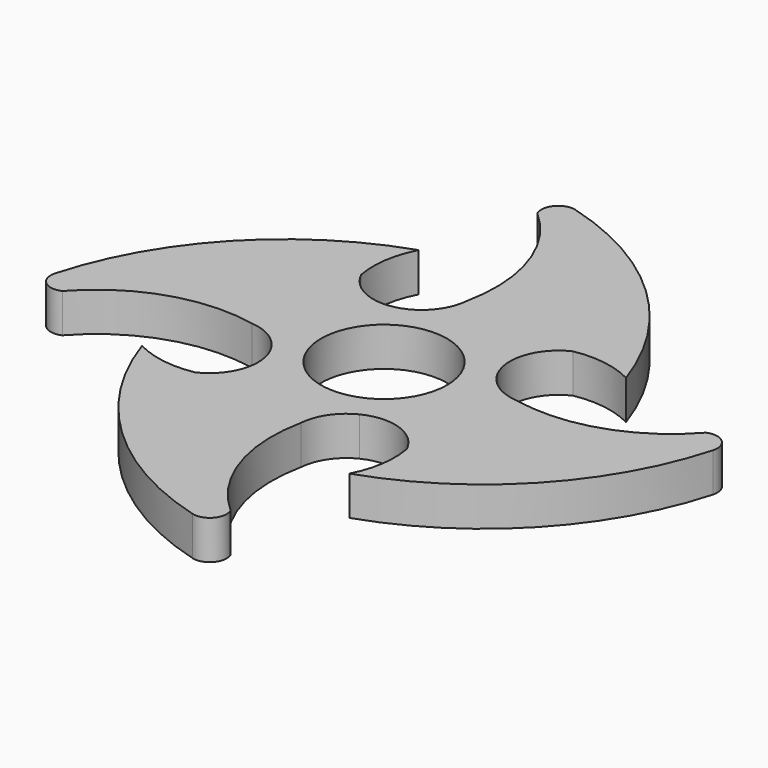
from build123d import *

# Parameters (mm, degrees)
F0_R        = 11.3
F1_DEPTH    = 7
F2_T1_DEPTH = 55.4992808982


# Not quite as in the source:
# - a fillet or chamfer that OpenCascade refuses, or shapes differently, is made with other operations: its cross-section is extruded or revolved along the edge and cut away or added
# - a feature names something its author has since deleted; it is built from what else it names


with BuildPart() as f1:
    # F0 (on Top) → F1 (new body)
    with BuildSketch(Plane.XY):
        with BuildLine():
            ThreePointArc((-19.0188516855, 18.6660698042), (-19.106601179, 24.2218879742), (-17.3798078978, 29.5032704141))
            ThreePointArc((-17.3798078978, 29.5032704141), (-42.8794362662, 11.5553714496), (-54.5032704141, -17.3798078978))
            ThreePointArc((-54.5032704141, -17.3798078978), (-51.6509498036, -14.2819027835), (-48.6055213036, -11.3736190606))
            ThreePointArc((-48.6055213036, -11.3736190606), (-36.3546417903, -3.2999675651), (-21.7060170396, -2.4719034169))
            ThreePointArc((-21.7060170396, -2.4719034169), (-17.5157178103, -3.9318400494), (-14.5899419176, -7.2679842351))
            ThreePointArc((-14.5899419176, -7.2679842351), (-15.4558877949, 5.1774059597), (-7.2679841768, 14.5899419466))
            ThreePointArc((-7.2679841768, 14.5899419466), (-14.000366861, 14.1575501664), (-19.0188516855, 18.6660698042))
        make_face()
        with BuildLine():
            ThreePointArc((-2.4719034169, 21.7060170396), (-3.9318400312, 17.5157178373), (-7.2679841768, 14.5899419466))
            ThreePointArc((-7.2679841768, 14.5899419466), (5.177405829, 15.4558878387), (14.5899417947, 7.2679844819))
            ThreePointArc((14.5899417947, 7.2679844819), (14.1575502222, 14.000367022), (18.6660698042, 19.0188516855))
            ThreePointArc((18.6660698042, 19.0188516855), (24.2218879742, 19.106601179), (29.5032704141, 17.3798078978))
            ThreePointArc((29.5032704141, 17.3798078978), (11.5553714496, 42.8794362662), (-17.3798078978, 54.5032704141))
            ThreePointArc((-17.3798078978, 54.5032704141), (-14.2819027835, 51.6509498036), (-11.3736190606, 48.6055213036))
            ThreePointArc((-11.3736190606, 48.6055213036), (-3.2999675651, 36.3546417903), (-2.4719034169, 21.7060170396))
        make_face()
        with BuildLine():
            ThreePointArc((14.5899417947, 7.2679844819), (5.177405829, 15.4558878387), (-7.2679841768, 14.5899419466))
            ThreePointArc((-7.2679841768, 14.5899419466), (-15.4558877949, 5.1774059597), (-14.5899419176, -7.2679842351))
            ThreePointArc((-14.5899419176, -7.2679842351), (-5.1774060707, -15.4558877577), (7.2679839673, -14.589942051))
            ThreePointArc((7.2679839673, -14.589942051), (13.8592593357, -8.5796812684), (16.3, 0))
            ThreePointArc((16.3, 0), (15.8667269979, 3.733225733), (14.5899417947, 7.2679844819))
        make_face()
        Circle(F0_R, mode=Mode.SUBTRACT)
        with BuildLine():
            ThreePointArc((7.2679839673, -14.589942051), (-5.1774060707, -15.4558877577), (-14.5899419176, -7.2679842351))
            ThreePointArc((-14.5899419176, -7.2679842351), (-14.157550177, -14.0003668918), (-18.6660698042, -19.0188516855))
            ThreePointArc((-18.6660698042, -19.0188516855), (-24.2218879742, -19.106601179), (-29.5032704141, -17.3798078978))
            ThreePointArc((-29.5032704141, -17.3798078978), (-11.5553714496, -42.8794362662), (17.3798078978, -54.5032704141))
            ThreePointArc((17.3798078978, -54.5032704141), (14.2819027835, -51.6509498036), (11.3736190606, -48.6055213036))
            ThreePointArc((11.3736190606, -48.6055213036), (3.2999675651, -36.3546417903), (2.4719034169, -21.7060170396))
            ThreePointArc((2.4719034169, -21.7060170396), (3.9318399658, -17.5157179344), (7.2679839673, -14.589942051))
        make_face()
        with BuildLine():
            ThreePointArc((21.7060170396, 2.4719034169), (17.515717696, 3.9318401265), (14.5899417947, 7.2679844819))
            ThreePointArc((14.5899417947, 7.2679844819), (15.8667269979, 3.733225733), (16.3, 0))
            ThreePointArc((16.3, 0), (13.8592593357, -8.5796812684), (7.2679839673, -14.589942051))
            ThreePointArc((7.2679839673, -14.589942051), (14.0003667504, -14.157550128), (19.0188516855, -18.6660698042))
            ThreePointArc((19.0188516855, -18.6660698042), (19.106601179, -24.2218879742), (17.3798078978, -29.5032704141))
            ThreePointArc((17.3798078978, -29.5032704141), (42.8794362662, -11.5553714496), (54.5032704141, 17.3798078978))
            ThreePointArc((54.5032704141, 17.3798078978), (51.6509498036, 14.2819027835), (48.6055213036, 11.3736190606))
            ThreePointArc((48.6055213036, 11.3736190606), (36.3546417903, 3.2999675651), (21.7060170396, 2.4719034169))
        make_face()
    extrude(amount=F1_DEPTH)

    # F2: fillet of radius 3 on 4 edges, made by hand

    # F2_s2 → F2_t1 (cut)
    with BuildSketch(Plane.XY.offset(-24.2496404491)):
        with BuildLine():
            ThreePointArc((-52.7416075724, -7.8412674467), (-51.7993975119, -10.9256989731), (-48.6055213036, -11.3736190606))
            ThreePointArc((-48.6055213036, -11.3736190606), (-51.6509498036, -14.2819027835), (-54.5032704141, -17.3798078978))
            ThreePointArc((-54.5032704141, -17.3798078978), (-53.8333652751, -12.5715819227), (-52.7416075724, -7.8412674467))
        make_face()
        with BuildLine():
            ThreePointArc((7.8412674467, -52.7416075724), (10.9256989731, -51.7993975119), (11.3736190606, -48.6055213036))
            ThreePointArc((11.3736190606, -48.6055213036), (14.2819027835, -51.6509498036), (17.3798078978, -54.5032704141))
            ThreePointArc((17.3798078978, -54.5032704141), (12.5715819227, -53.8333652751), (7.8412674467, -52.7416075724))
        make_face()
        with BuildLine():
            ThreePointArc((52.7416075724, 7.8412674467), (51.7993975119, 10.9256989731), (48.6055213036, 11.3736190606))
            ThreePointArc((48.6055213036, 11.3736190606), (51.6509498036, 14.2819027835), (54.5032704141, 17.3798078978))
            ThreePointArc((54.5032704141, 17.3798078978), (53.8333652751, 12.5715819227), (52.7416075724, 7.8412674467))
        make_face()
        with BuildLine():
            ThreePointArc((-7.8412674467, 52.7416075724), (-10.9256989731, 51.7993975119), (-11.3736190606, 48.6055213036))
            ThreePointArc((-11.3736190606, 48.6055213036), (-14.2819027835, 51.6509498036), (-17.3798078978, 54.5032704141))
            ThreePointArc((-17.3798078978, 54.5032704141), (-12.5715819227, 53.8333652751), (-7.8412674467, 52.7416075724))
        make_face()
    extrude(amount=F2_T1_DEPTH, mode=Mode.SUBTRACT)


solid = f1.part
